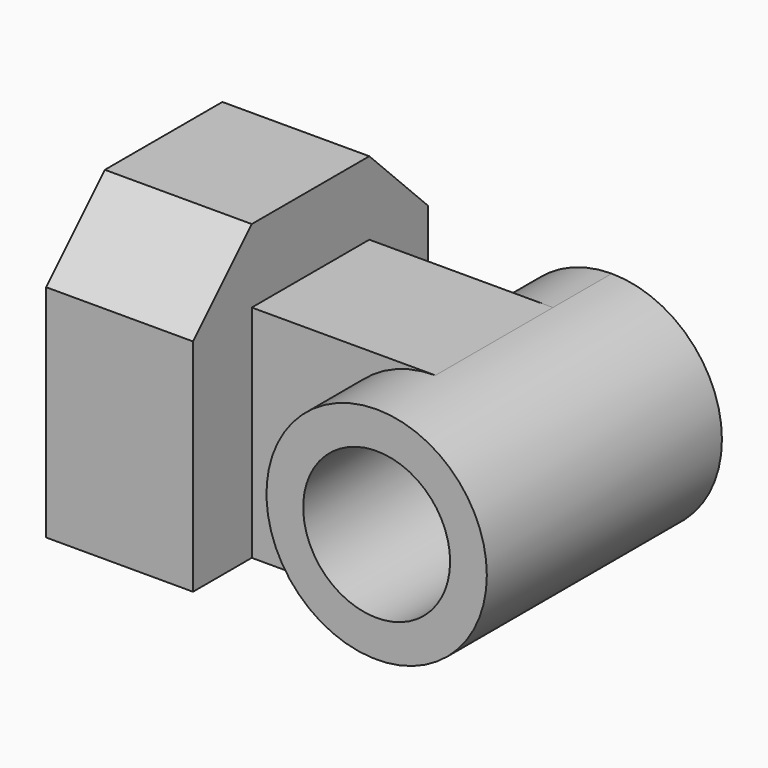
from build123d import *

# Parameters (mm, degrees)
F0_W     = 38.1
F0_H     = 25.4
F1_DEPTH = 25.4
F3_DEPTH = 12.7
F5_DEPTH = 25.4
F6_DEPTH = 6.35
F4_R     = 6.35
F7_DEPTH = 25.4
F9_DEPTH = 6.35


with BuildPart() as f1:
    # F0 (on Top) → F1 (new body)
    with BuildSketch(Plane.XY):
        with Locations((19.05, 12.7)):
            Rectangle(F0_W, F0_H)
    extrude(amount=F1_DEPTH)

    # F2 (on face) → F3 (cut)
    with BuildSketch(Plane(origin=(0, 0, 0), x_dir=(0, -1, 0), z_dir=(-1, 0, 0))):
        Polygon((-19.05, 25.4), (-25.4, 25.4), (-25.4, 19.05), align=None)
        Polygon((0, 19.05), (0, 25.4), (-6.35, 25.4), align=None)
    extrude(amount=-F3_DEPTH, mode=Mode.SUBTRACT)

    # F4 (on face) → F5 (cut)
    with BuildSketch(Plane.XZ):
        with BuildLine():
            ThreePointArc((28.575, 19.05), (35.3101920908, 16.2601920908), (38.1, 9.525))
            Line((38.1, 9.525), (38.1, 25.4))
            Line((38.1, 25.4), (12.7, 25.4))
            Line((12.7, 25.4), (12.7, 19.05))
            Line((12.7, 19.05), (28.575, 19.05))
        make_face()
        with BuildLine():
            Line((38.1, 0), (38.1, 9.525))
            ThreePointArc((38.1, 9.525), (35.3101920908, 2.7898079092), (28.575, 0))
            Line((28.575, 0), (38.1, 0))
        make_face()
    extrude(amount=-F5_DEPTH, mode=Mode.SUBTRACT)

    # F4 (on face) → F6 (cut)
    with BuildSketch(Plane.XZ):
        with BuildLine():
            ThreePointArc((28.575, 0), (19.05, 9.525), (28.575, 19.05))
            Line((28.575, 19.05), (12.7, 19.05))
            Line((12.7, 19.05), (12.7, 0))
            Line((12.7, 0), (28.575, 0))
        make_face()
    extrude(amount=-F6_DEPTH, mode=Mode.SUBTRACT)

    # F4 (on face) → F7 (cut)
    with BuildSketch(Plane.XZ):
        with Locations((28.575, 9.525)):
            Circle(F4_R)
    extrude(amount=-F7_DEPTH, mode=Mode.SUBTRACT)

    # F8 (on face) → F9 (cut)
    with BuildSketch(Plane(origin=(0, 25.4, 0), x_dir=(-1, 0, 0), z_dir=(0, 1, 0))):
        with BuildLine():
            ThreePointArc((-28.575, 19.05), (-21.8398079092, 16.2601920908), (-19.05, 9.525))
            ThreePointArc((-19.05, 9.525), (-21.8398079092, 2.7898079092), (-28.575, 0))
            Line((-28.575, 0), (-12.7, 0))
            Line((-12.7, 0), (-12.7, 19.05))
            Line((-12.7, 19.05), (-28.575, 19.05))
        make_face()
    extrude(amount=-F9_DEPTH, mode=Mode.SUBTRACT)


solid = f1.part
